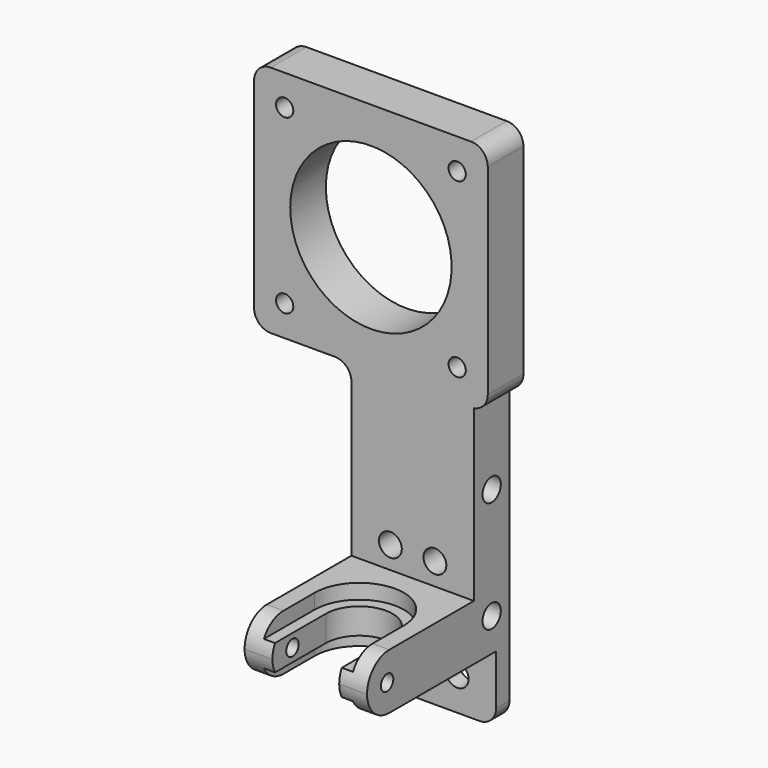
from build123d import *

# Parameters (mm, degrees)
F0_W          = 22
F0_H          = 42
F1_DEPTH      = 3
F2_W          = 3
F2_H          = 30
F2_W_2        = 5
F3_DEPTH      = 22
F4_D          = 4.1
F7_DEPTH      = 5
F8_DEPTH      = 2.325
F9_R          = 4.99999
F11_D         = 4.1
F12_D         = 2.8
F13_W         = 22
F13_H         = 10.5
F14_DEPTH     = 8
F15_T1_DEPTH  = 8
F15_T3_DEPTH  = 18
F15_T5_DEPTH  = 18
F15_T7_DEPTH  = 22.7901994578
F15_T9_DEPTH  = 23
F15_T11_DEPTH = 23
F15_T13_DEPTH = 23
F16_D         = 29
F17_D         = 3.1


# Not quite as in the source:
# - a fillet or chamfer that OpenCascade refuses, or shapes differently, is made with other operations: its cross-section is extruded or revolved along the edge and cut away or added
# - a fillet or chamfer is up to 0.001 mm smaller than in the source, because OpenCascade refuses the exact size


with BuildPart() as f1:
    # F0 (on Front) → F1 (new body)
    with BuildSketch(Plane.XZ):
        with Locations((-28.9233987555, 27.9422005266)):
            Rectangle(F0_W, F0_H)
    extrude(amount=F1_DEPTH)

    # F2 (on face) → F3 (join)
    with BuildSketch(Plane(origin=(-39.9233987555, 0, 0), x_dir=(0, -1, 0), z_dir=(-1, 0, 0))):
        with Locations((1.5, 33.9422005266)):
            Rectangle(F2_W, F2_H)
        with Locations((5.5, 33.9422005266)):
            Rectangle(F2_W_2, F2_H)
    extrude(amount=-F3_DEPTH)

    # F4 (through all)
    with Locations(Plane(origin=(0, 0, 0), x_dir=(1, 0, 0), z_dir=(0, 1, 0))):
        with Locations((-24.9233987555, -12.9422005266), (-32.9233987555, -12.9422005266), (-32.9233987555, -32.9422005266), (-24.9233987555, -32.9422005266)):
            Hole(F4_D / 2)

    # F6 (on line) → F7 (join, symmetric)
    with BuildSketch(Plane.XY.offset(23.9422005266)):
        with BuildLine():
            ThreePointArc((-36.9233987555, -20), (-28.9233987555, -12), (-20.9233987555, -20))
            Line((-20.9233987555, -20), (-20.9233987555, -32))
            Line((-20.9233987555, -32), (-17.9233987555, -32))
            Line((-17.9233987555, -32), (-17.9233987555, 0))
            Line((-17.9233987555, 0), (-39.9233987555, 0))
            Line((-39.9233987555, 0), (-39.9233987555, -32))
            Line((-39.9233987555, -32), (-36.9233987555, -32))
            Line((-36.9233987555, -32), (-36.9233987555, -20))
        make_face()
    extrude(amount=F7_DEPTH, both=True)

    # F6 (on line) → F8 (join, symmetric)
    with BuildSketch(Plane.XY.offset(23.9422005266)):
        with BuildLine():
            ThreePointArc((-34.9233987555, -20), (-28.9233987555, -14), (-22.9233987555, -20))
            Line((-22.9233987555, -20), (-22.9233987555, -25.2915026221))
            ThreePointArc((-22.9233987555, -25.2915026221), (-21.4400839819, -22.8284271247), (-20.9233987555, -20))
            ThreePointArc((-20.9233987555, -20), (-28.9233987555, -12), (-36.9233987555, -20))
            ThreePointArc((-36.9233987555, -20), (-36.406713529, -22.8284271247), (-34.9233987555, -25.2915026221))
            Line((-34.9233987555, -25.2915026221), (-34.9233987555, -20))
        make_face()
        with BuildLine():
            Line((-34.9233987555, -32), (-34.9233987555, -25.2915026221))
            ThreePointArc((-34.9233987555, -25.2915026221), (-36.406713529, -22.8284271247), (-36.9233987555, -20))
            Line((-36.9233987555, -20), (-36.9233987555, -32))
            Line((-36.9233987555, -32), (-34.9233987555, -32))
        make_face()
        with BuildLine():
            ThreePointArc((-20.9233987555, -20), (-21.4400839819, -22.8284271247), (-22.9233987555, -25.2915026221))
            Line((-22.9233987555, -25.2915026221), (-22.9233987555, -32))
            Line((-22.9233987555, -32), (-20.9233987555, -32))
            Line((-20.9233987555, -32), (-20.9233987555, -20))
        make_face()
    extrude(amount=F8_DEPTH, both=True)

    # F9 (radius 5 in the source; OpenCascade refuses exactly that, so slightly less here)
    f9_edges = [f1.edges().sort_by_distance(p)[0] for p in [
        (-38.423399, -32, 28.942201),
        (-38.423399, -32, 18.942201),
        (-19.423399, -32, 18.942201),
        (-19.423399, -32, 28.942201),
    ]]
    fillet(f9_edges, radius=F9_R)

    # F11 (through all)
    with Locations(Plane(origin=(-39.9233987555, 0, 0), x_dir=(0, -1, 0), z_dir=(-1, 0, 0))):
        with Locations((4, 44.9422005266), (4, 24.9422005266)):
            Hole(F11_D / 2)

    # F12 (through all)
    with Locations(Plane(origin=(-39.9233987555, 0, 0), x_dir=(0, -1, 0), z_dir=(-1, 0, 0))):
        with Locations((27.5, 23.9422005266)):
            Hole(F12_D / 2)

    # F13 (on Front) → F14 (join)
    with BuildSketch(Plane.XZ):
        Polygon((-57.4233987555, 59.4422005266), (-39.9233987555, 59.4422005266), (-17.9233987555, 59.4422005266), (-15.4233987555, 59.4422005266), (-15.4233987555, 101.4422005266), (-57.4233987555, 101.4422005266), align=None)
        with Locations((-28.9233987555, 54.1922005266)):
            Rectangle(F13_W, F13_H)
    extrude(amount=F14_DEPTH)

    # F15: fillet of radius 3 on 7 edges, made by hand

    # F15_s2 → F15_t1 (join)
    with BuildSketch(Plane.XZ):
        with BuildLine():
            ThreePointArc((-39.9233987555, 56.4422005266), (-40.8020784119, 58.5635208702), (-42.9233987555, 59.4422005266))
            Line((-42.9233987555, 59.4422005266), (-39.9233987555, 59.4422005266))
            Line((-39.9233987555, 59.4422005266), (-39.9233987555, 56.4422005266))
        make_face()
    extrude(amount=F15_T1_DEPTH)

    # F15_s4 → F15_t3 (cut)
    with BuildSketch(Plane.XZ.offset(-7.5)):
        with BuildLine():
            ThreePointArc((-39.9233987555, 9.9422005266), (-39.0447190991, 7.820880183), (-36.9233987555, 6.9422005266))
            Line((-36.9233987555, 6.9422005266), (-39.9233987555, 6.9422005266))
            Line((-39.9233987555, 6.9422005266), (-39.9233987555, 9.9422005266))
        make_face()
    extrude(amount=F15_T3_DEPTH, mode=Mode.SUBTRACT)

    # F15_s6 → F15_t5 (cut)
    with BuildSketch(Plane.XZ.offset(-7.5)):
        with BuildLine():
            ThreePointArc((-17.9233987555, 9.9422005266), (-18.8020784119, 7.820880183), (-20.9233987555, 6.9422005266))
            Line((-20.9233987555, 6.9422005266), (-17.9233987555, 6.9422005266))
            Line((-17.9233987555, 6.9422005266), (-17.9233987555, 9.9422005266))
        make_face()
    extrude(amount=F15_T5_DEPTH, mode=Mode.SUBTRACT)

    # F15_s8 → F15_t7 (cut)
    with BuildSketch(Plane.XZ.offset(-7.3950997289)):
        with BuildLine():
            ThreePointArc((-17.9233987555, 59.4422005266), (-16.132110908, 60.463748745), (-15.4233987555, 62.4002404181))
            Line((-15.4233987555, 62.4002404181), (-15.4233987555, 59.4422005266))
            Line((-15.4233987555, 59.4422005266), (-17.9233987555, 59.4422005266))
        make_face()
    extrude(amount=F15_T7_DEPTH, mode=Mode.SUBTRACT)

    # F15_s10 → F15_t9 (cut)
    with BuildSketch(Plane.XZ.offset(-7.5)):
        with BuildLine():
            ThreePointArc((-18.4233987555, 101.4422005266), (-16.3020784119, 100.5635208702), (-15.4233987555, 98.4422005266))
            Line((-15.4233987555, 98.4422005266), (-15.4233987555, 101.4422005266))
            Line((-15.4233987555, 101.4422005266), (-18.4233987555, 101.4422005266))
        make_face()
    extrude(amount=F15_T9_DEPTH, mode=Mode.SUBTRACT)

    # F15_s12 → F15_t11 (cut)
    with BuildSketch(Plane.XZ.offset(-7.5)):
        with BuildLine():
            ThreePointArc((-57.4233987555, 98.4422005266), (-56.5447190991, 100.5635208702), (-54.4233987555, 101.4422005266))
            Line((-54.4233987555, 101.4422005266), (-57.4233987555, 101.4422005266))
            Line((-57.4233987555, 101.4422005266), (-57.4233987555, 98.4422005266))
        make_face()
    extrude(amount=F15_T11_DEPTH, mode=Mode.SUBTRACT)

    # F15_s14 → F15_t13 (cut)
    with BuildSketch(Plane.XZ.offset(-7.5)):
        with BuildLine():
            ThreePointArc((-54.4233987555, 59.4422005266), (-56.5447190991, 60.320880183), (-57.4233987555, 62.4422005266))
            Line((-57.4233987555, 62.4422005266), (-57.4233987555, 59.4422005266))
            Line((-57.4233987555, 59.4422005266), (-54.4233987555, 59.4422005266))
        make_face()
    extrude(amount=F15_T13_DEPTH, mode=Mode.SUBTRACT)

    # F16 (through all)
    with Locations(Plane(origin=(0, 0, 0), x_dir=(1, 0, 0), z_dir=(0, 1, 0))):
        with Locations((-36.4233987555, -80.4422005266)):
            Hole(F16_D / 2)

    # F17 (through all)
    with Locations(Plane(origin=(0, 0, 0), x_dir=(1, 0, 0), z_dir=(0, 1, 0))):
        with Locations((-51.9233987555, -95.9422005266), (-20.9233987555, -95.9422005266), (-20.9233987555, -64.9422005266), (-51.9233987555, -64.9422005266)):
            Hole(F17_D / 2)


solid = f1.part
